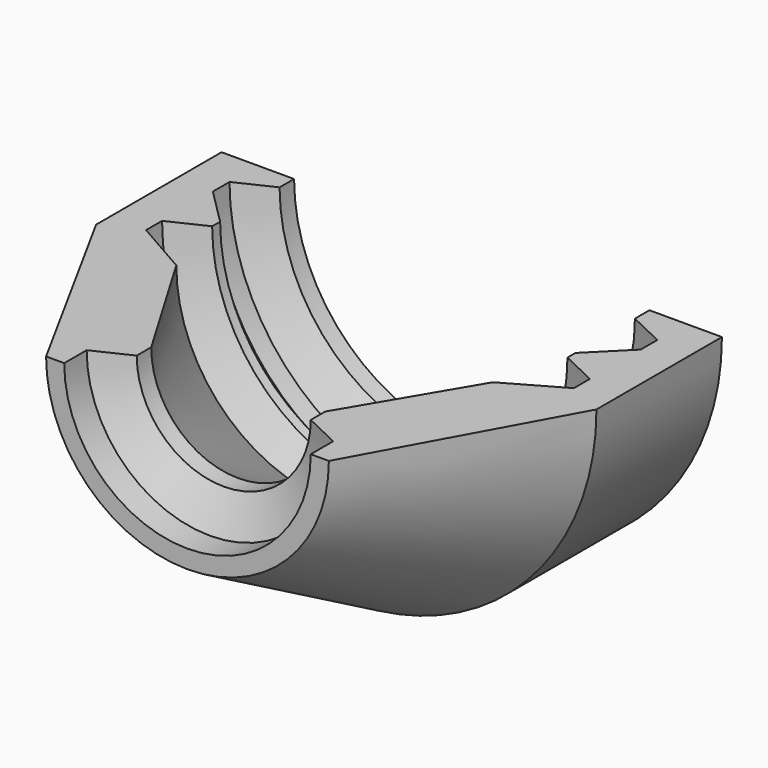
from build123d import *

# Parameters (mm, degrees)
F1_ANGLE    = 180
F2_T4_ANGLE = 243.6352501502
F2_S5_R     = 11.8
F2_T6_DEPTH = 16
F3_T4_ANGLE = 243.2500896942
F3_S5_R     = 11.8
F3_T6_DEPTH = 16
F4_T4_ANGLE = 243.7164036037
F4_S5_R     = 11.8
F4_T6_DEPTH = 16
F5_T4_ANGLE = 243.7164036037
F5_S5_R     = 11.8
F5_T6_DEPTH = 16
F6_T4_ANGLE = 310.0876573575
F6_S5_R     = 6.8
F6_T6_DEPTH = 11


# Not quite as in the source:
# - a fillet or chamfer that OpenCascade refuses, or shapes differently, is made with other operations: its cross-section is extruded or revolved along the edge and cut away or added


with BuildPart() as f1:
    # F0 (on Top) → F1 (revolve)
    with BuildSketch(Plane.XY):
        Polygon((-11.8, 5.65), (-11.8, 6.65), (-13.8, 6.65), (-13.8, 0), (-7.8, -10.95), (-6.8, -10.95), (-6.8, -9.45), (-4.8, -9.45), (-4.8, -7.45), (-9.8, 1), (-11.8, 1), (-11.8, 2), (-9.8, 2), (-9.8, 5.65), align=None)
        Polygon((-13.8, 6.65), (-11.8, 6.65), (-9.8, 6.65), (-9.8, 8.65), (-13.8, 8.65), align=None)
    revolve(axis=Axis((0, 0, 0), (0, -1, 0)), revolution_arc=F1_ANGLE)

    # F2: chamfer of 2.1 on 1 edges, made by hand


with BuildPart() as f2_tool2:
    # F2_s3 → F2_t4 (revolve)
    with BuildSketch(Plane(origin=(0, 0, 0), x_dir=(0, 1, 0), z_dir=(0.5272172108, 0, 0.849730553))):
        Polygon((-0.8073066866, 8.7305877594), (1, 11.9), (1, 9.8), align=None)
    revolve(axis=Axis((0, 1, 0), (0, -1, 0)), revolution_arc=F2_T4_ANGLE)

    # F2_s5 → F2_t6 (intersect, symmetric)
    with BuildSketch(Plane.XZ.offset(-0.1)):
        Circle(F2_S5_R)
    extrude(amount=F2_T6_DEPTH, both=True, mode=Mode.INTERSECT)


with BuildPart() as f1_1:
    add(f1.part)

    # F2_t1: cut F2_tool2
    add(f2_tool2.part, mode=Mode.SUBTRACT)

    # F3: chamfer of 2.1 on 1 edges, made by hand


with BuildPart() as f3_tool2:
    # F3_s3 → F3_t4 (revolve)
    with BuildSketch(Plane(origin=(0, 0, 0), x_dir=(0, 1, 0), z_dir=(0.5243581586, 0, 0.8514978107))):
        Polygon((5.65, 11.9), (3.55, 9.8), (5.65, 9.8), align=None)
    revolve(axis=Axis((0, 5.65, 0), (0, -1, 0)), revolution_arc=F3_T4_ANGLE)

    # F3_s5 → F3_t6 (intersect, symmetric)
    with BuildSketch(Plane.XZ.offset(-4.6)):
        Circle(F3_S5_R)
    extrude(amount=F3_T6_DEPTH, both=True, mode=Mode.INTERSECT)


with BuildPart() as f1_2:
    add(f1_1.part)

    # F3_t1: cut F3_tool2
    add(f3_tool2.part, mode=Mode.SUBTRACT)

    # F4: chamfer of 2.1 x 1 on 1 edges, made by hand


with BuildPart() as f4_tool2:
    # F4_s3 → F4_t4 (revolve)
    with BuildSketch(Plane(origin=(0, 0, 0), x_dir=(0, 1, 0), z_dir=(0.5278188556, 0, 0.849356966))):
        Polygon((7.65, 9.8), (6.65, 11.9), (6.65, 9.8), align=None)
    revolve(axis=Axis((0, 6.65, 0), (0, -1, 0)), revolution_arc=F4_T4_ANGLE)

    # F4_s5 → F4_t6 (intersect, symmetric)
    with BuildSketch(Plane.XZ.offset(-7.2)):
        Circle(F4_S5_R)
    extrude(amount=F4_T6_DEPTH, both=True, mode=Mode.INTERSECT)


with BuildPart() as f1_3:
    add(f1_2.part)

    # F4_t1: cut F4_tool2
    add(f4_tool2.part, mode=Mode.SUBTRACT)

    # F5: chamfer of 2.1 x 1 on 1 edges, made by hand


with BuildPart() as f5_tool2:
    # F5_s3 → F5_t4 (revolve)
    with BuildSketch(Plane(origin=(0, 0, 0), x_dir=(0, 1, 0), z_dir=(0.5278188556, 0, 0.849356966))):
        Polygon((3, 9.8), (2, 11.9), (2, 9.8), align=None)
    revolve(axis=Axis((0, 2, 0), (0, -1, 0)), revolution_arc=F5_T4_ANGLE)

    # F5_s5 → F5_t6 (intersect, symmetric)
    with BuildSketch(Plane.XZ.offset(-2.5)):
        Circle(F5_S5_R)
    extrude(amount=F5_T6_DEPTH, both=True, mode=Mode.INTERSECT)


with BuildPart() as f1_4:
    add(f1_3.part)

    # F5_t1: cut F5_tool2
    add(f5_tool2.part, mode=Mode.SUBTRACT)

    # F6: chamfer of 2.1 x 1 on 1 edges, made by hand


with BuildPart() as f6_tool2:
    # F6_s3 → F6_t4 (revolve)
    with BuildSketch(Plane(origin=(0, 0, 0), x_dir=(0, 1, 0), z_dir=(0.9066308057, 0, 0.4219248537))):
        Polygon((-8.45, 4.8), (-9.45, 6.9), (-9.45, 4.8), align=None)
    revolve(axis=Axis((0, -9.45, 0), (0, -1, 0)), revolution_arc=F6_T4_ANGLE)

    # F6_s5 → F6_t6 (intersect, symmetric)
    with BuildSketch(Plane.XZ.offset(8.9)):
        Circle(F6_S5_R)
    extrude(amount=F6_T6_DEPTH, both=True, mode=Mode.INTERSECT)


with BuildPart() as f1_5:
    add(f1_4.part)

    # F6_t1: cut F6_tool2
    add(f6_tool2.part, mode=Mode.SUBTRACT)


solid = f1_5.part
